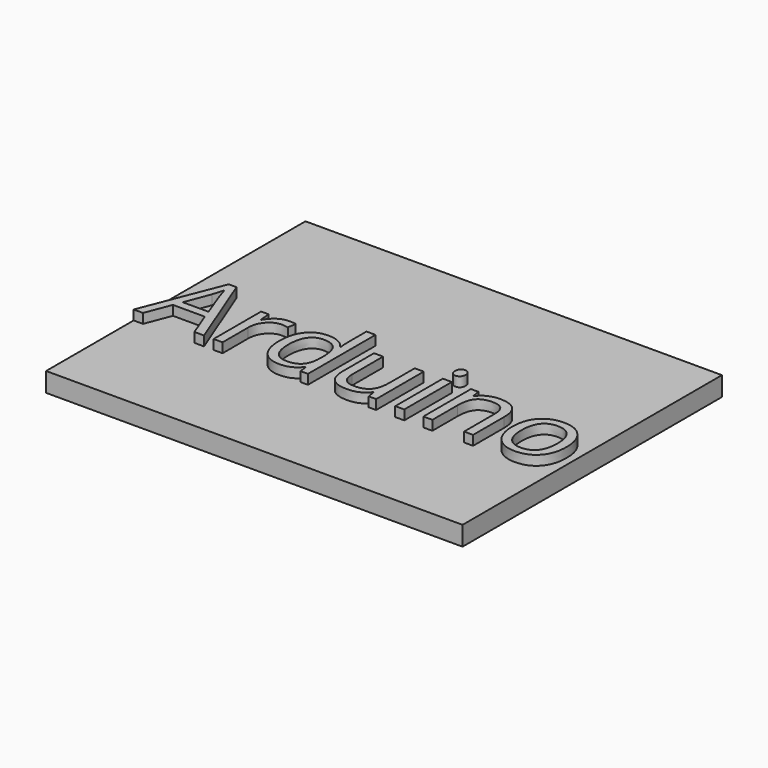
from build123d import *

# Parameters (mm, degrees)
F0_W         = 68.6
F0_H         = 53.4
F1_DEPTH     = 3.175
F2_TEXT_SIZE = 18.3078270297
F3_DEPTH     = 1.5875


# Not quite as in the source:
# - Text() gives the source's letters only with a copy of the font that has no kerning and outlines rounded to 1/6400 em; it was checked with that copy


with BuildPart() as f1:
    # F0 (on Top) → F1 (new body)
    with BuildSketch(Plane.XY):
        Rectangle(F0_W, F0_H)
    extrude(amount=F1_DEPTH)

    # F2 (on face) → F3 (join)
    with BuildSketch(Plane.XY.offset(3.175)):
        with Locations((-34.3, -8.670219004)):
            Text('Arduino', F2_TEXT_SIZE, font='Open Sans', text_align=(TextAlign.LEFT, TextAlign.BOTTOM))
    extrude(amount=F3_DEPTH)


solid = f1.part
